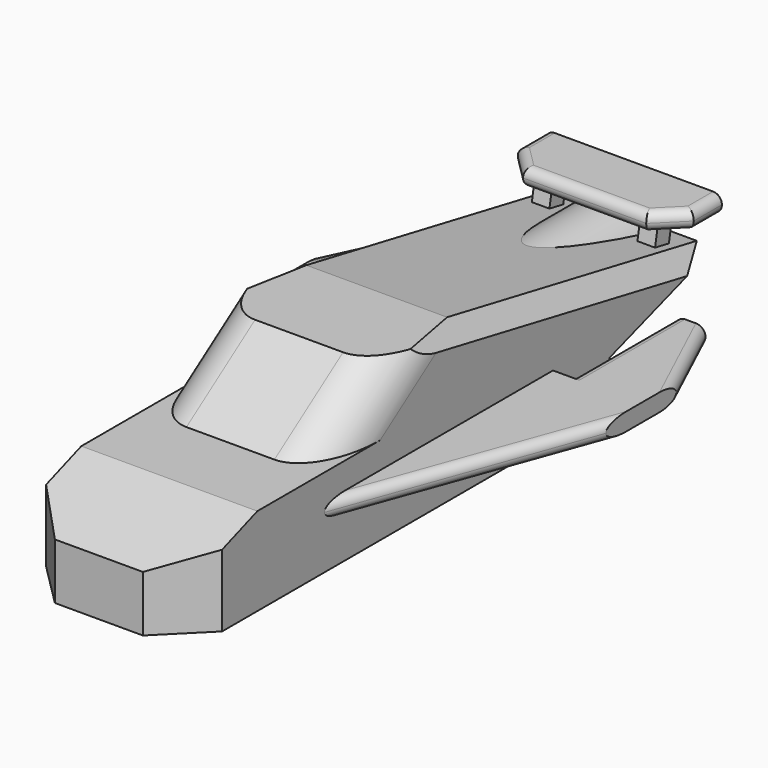
from build123d import *

# Parameters (mm, degrees)
F1_DEPTH     = 10
F2_DEPTH     = 10
F3_R         = 5
F4_T1_DEPTH  = 71.883894651
F5_T1_DEPTH  = 56.6843134125
F6_SIZE      = 3
F7_SIZE      = 5
F10_DEPTH    = 10
F9_W         = 35
F9_H         = 2
F11_DEPTH    = 10
F12_T4_DEPTH = 157.651683953
F13_T4_DEPTH = 157.651683953
F14_W        = 8
F14_H        = 2
F15_W        = 8
F15_H        = 2
F16_DEPTH    = 15
F17_SIZE2    = 4.6630765815
F17_SIZE     = 10
F18_SIZE2    = 4.6630765815
F18_SIZE     = 10
F19_R        = 0.99999
F20_R        = 5
F21_DEPTH    = 45
F22_R        = 2.9781353661
F23_DEPTH    = 5
F25_W        = 2
F25_H        = 2
F26_DEPTH    = 4
F28_DEPTH    = 15
F29_DEPTH    = 5
F30_W        = 5
F30_H        = 2
F31_DEPTH    = 2
F32_SIZE     = 3
F33_R        = 0.99999


# Not quite as in the source:
# - a fillet or chamfer that OpenCascade refuses, or shapes differently, is made with other operations: its cross-section is extruded or revolved along the edge and cut away or added
# - a fillet or chamfer is up to 0.001 mm smaller than in the source, because OpenCascade refuses the exact size


with BuildPart() as f1:
    # F0 (on Right) → F1 (new body)
    with BuildSketch(Plane.YZ):
        Polygon((30, 5), (30, 0), (44.9290536344, 5), (9.4593074173, 11.7742568254), (-1.5650746645, 11.7742568254), (-11.31126564, 5), align=None)
        Polygon((30, 0), (0, 0), (-30, 0), (-30, -5), (30, -5), align=None)
        Polygon((-30, 0), (0, 0), (30, 0), (30, 5), (-11.31126564, 5), (-30, 5), align=None)
    extrude(amount=-F1_DEPTH)

    # F2 (add): a face of the model
    f2_faces = [f1.faces().sort_by_distance(p)[0] for p in [
        (0, 4.6213303299, 2.1526362718),
    ]]
    extrude(f2_faces, amount=F2_DEPTH)

    # F3
    f3_edges = [f1.edges().sort_by_distance(p)[0] for p in [
        (-10, -6.43817, 8.387128),
        (10, -6.43817, 8.387128),
    ]]
    fillet(f3_edges, radius=F3_R)

    # F4: chamfer of 10 x 3.6397023427 on 1 edges, made by hand

    # F4_s2 → F4_t1 (cut)
    with BuildSketch(Plane.YZ.offset(-35.9419473255)):
        Polygon((-20, 5), (-30, 1.3602976573), (-30, 5), align=None)
    extrude(amount=F4_T1_DEPTH, mode=Mode.SUBTRACT)

    # F5: chamfer of 2 on 2 edges, made by hand

    # F5_s2 → F5_t1 (cut)
    with BuildSketch(Plane(origin=(0, 47.4786197454, -9.0677943367), x_dir=(1, 0, 0), z_dir=(0, -0.9822462418, 0.1875961634))):
        Polygon((-10, 11.3397492965), (-8, 13.3397492965), (-10, 13.3397492965), align=None)
        Polygon((10, 11.3397492965), (8, 13.3397492965), (10, 13.3397492965), align=None)
    extrude(amount=F5_T1_DEPTH, mode=Mode.SUBTRACT)

    # F6
    f6_edges = [f1.edges().sort_by_distance(p)[0] for p in [
        (0, 30, -5),
    ]]
    chamfer(f6_edges, length=F6_SIZE)

    # F7
    f7_edges = [f1.edges().sort_by_distance(p)[0] for p in [
        (-10, -30, -1.819851),
        (10, -30, -1.819851),
    ]]
    chamfer(f7_edges, length=F7_SIZE)

    # F8 (on face) → F10 (join)
    with BuildSketch(Plane.YZ.offset(10)):
        Polygon((-13, 0), (0, 0), (22, 0), (22, 2), (-13, 2), align=None)
    extrude(amount=F10_DEPTH)

    # F9 (on face) → F11 (join)
    with BuildSketch(Plane(origin=(-10, 0, 0), x_dir=(0, -1, 0), z_dir=(-1, 0, 0))):
        with Locations((-4.5269672573, 1)):
            Rectangle(F9_W, F9_H)
    extrude(amount=F11_DEPTH)

    # F12: chamfer of 30 x 10.919107028 on 1 edges, made by hand


with BuildPart() as f12_tool2:
    # F12_s3 → F12_t4 (new body)
    with BuildSketch(Plane.XY.offset(-77.8258419765)):
        Polygon((-9.080892972, -12.9730327427), (-20, 17.0269672573), (-20, -12.9730327427), align=None)
    extrude(amount=F12_T4_DEPTH)

    split(bisect_by=Plane.YZ.offset(-10), keep=Keep.BOTTOM)


with BuildPart() as f1_1:
    add(f1.part)

    # F12_t1: cut F12_tool2
    add(f12_tool2.part, mode=Mode.SUBTRACT)

    # F13: chamfer of 30 x 10.919107028 on 1 edges, made by hand


with BuildPart() as f13_tool2:
    # F13_s3 → F13_t4 (new body)
    with BuildSketch(Plane.XY.offset(79.8258419765)):
        Polygon((9.080892972, -13), (20, 17), (20, -13), align=None)
    extrude(amount=-F13_T4_DEPTH)

    split(bisect_by=Plane.YZ.offset(10), keep=Keep.TOP)


with BuildPart() as f1_2:
    add(f1_1.part)

    # F13_t1: cut F13_tool2
    add(f13_tool2.part, mode=Mode.SUBTRACT)

    # F14 (on face) + F15 (on face) → F16 (join)
    with BuildSketch(Plane(origin=(0, 22, 0), x_dir=(-1, 0, 0), z_dir=(0, 1, 0))):
        with Locations((-16, 1)):
            Rectangle(F14_W, F14_H)
    with BuildSketch(Plane(origin=(0, 22.0269672573, 0), x_dir=(-1, 0, 0), z_dir=(0, 1, 0))):
        with Locations((16, 1)):
            Rectangle(F15_W, F15_H)
    extrude(amount=F16_DEPTH)

    # F17
    f17_edges = [f1_2.edges().sort_by_distance(p)[0] for p in [
        (20, 37, 1),
    ]]
    f17_side = f1_2.faces().sort_by_distance((20, 27, 1))[0]
    chamfer(f17_edges, length=F17_SIZE, length2=F17_SIZE2, reference=f17_side)

    # F18
    f18_edges = [f1_2.edges().sort_by_distance(p)[0] for p in [
        (-20, 37.026967, 1),
    ]]
    f18_side = f1_2.faces().sort_by_distance((-20, 27.026967, 1))[0]
    chamfer(f18_edges, length=F18_SIZE, length2=F18_SIZE2, reference=f18_side)

    # F19 (radius 1 in the source; OpenCascade refuses exactly that, so slightly less here)
    f19_edges = [f1_2.edges().sort_by_distance(p)[0] for p in [
        (15, 3.262613, 2),
        (15, 3.262613, 0),
        (17.668462, 32, 0),
        (17.668462, 32, 2),
        (12, 29.5, 2),
        (12, 29.5, 0),
        (-15, 3.28958, 2),
        (-15, 3.28958, 0),
        (-17.668462, 32.026967, 2),
        (-12, 29.526967, 2),
        (-12, 29.526967, 0),
    ]]
    fillet(f19_edges, radius=F19_R)

    # F20 (on Front) → F21 (join)
    with BuildSketch(Plane.XZ):
        with Locations((0, 2.7116553392)):
            Circle(F20_R)
    extrude(amount=-F21_DEPTH)

    # F22 (on face) → F23 (cut)
    with BuildSketch(Plane(origin=(0, 45, 0), x_dir=(-1, 0, 0), z_dir=(0, 1, 0))):
        with Locations((0, 2.7116553392)):
            Circle(F22_R)
    extrude(amount=-F23_DEPTH, mode=Mode.SUBTRACT)

    # F24: chamfer of 2 on 1 edges, made by hand


with BuildPart() as f24_tool2:
    # F24_s3 → F24_t4 (revolve)
    with BuildSketch(Plane.XY.offset(2.7116553392)):
        Polygon((5, 43), (3, 45), (5, 45), align=None)
    revolve(axis=Axis((0, 45, 2.7116553392), (0, -1, 0)))

    split(bisect_by=Plane(origin=(0, 3.0256985599, -9.0341632165), x_dir=(1, 0, 0), z_dir=(0, 0.3175793108, -0.9482317129)), keep=Keep.TOP)


with BuildPart() as f1_3:
    add(f1_2.part)

    # F24_t1: cut F24_tool2
    add(f24_tool2.part, mode=Mode.SUBTRACT)


with BuildPart() as f24_tool7:
    # F24_s8 → F24_t9 (revolve)
    with BuildSketch(Plane.XY.offset(2.7116553392)):
        Polygon((5, 43), (3, 45), (5, 45), align=None)
    revolve(axis=Axis((0, 45, 2.7116553392), (0, -1, 0)))

    split(bisect_by=Plane(origin=(0, 2.5024857889, 13.1029186126), x_dir=(1, 0, 0), z_dir=(0, 0.1875961634, 0.9822462418)), keep=Keep.TOP)


with BuildPart() as f1_4:
    add(f1_3.part)

    # F24_t6: cut F24_tool7
    add(f24_tool7.part, mode=Mode.SUBTRACT)

    # F25 (on face) → F26 (join)
    with BuildSketch(Plane(origin=(0, 2.5024857889, 13.1029186126), x_dir=(1, 0, 0), z_dir=(0, 0.1875961634, 0.9822462418))):
        with Locations((-6, 39.4243540466)):
            Rectangle(F25_W, F25_H)
        with Locations((6, 39.4243540466)):
            Rectangle(F25_W, F25_H)
    extrude(amount=F26_DEPTH)

    # F27 (on face) → F28 (join)
    with BuildSketch(Plane(origin=(5, 0, 0), x_dir=(0, -1, 0), z_dir=(-1, 0, 0))):
        Polygon((-42.9595402808, 9.4484498521), (-40.9950477973, 9.8236421789), (-45.9950477973, 9.8236421789), (-45.9950477973, 7.8236421789), (-42.6492233025, 7.8236421789), align=None)
        Polygon((-40.9950477973, 7.8236421789), (-40.9950477973, 9.8236421789), (-42.9595402808, 9.4484498521), (-42.6492233025, 7.8236421789), align=None)
    extrude(amount=F28_DEPTH)

    # F27 (on face) → F29 (join)
    with BuildSketch(Plane(origin=(5, 0, 0), x_dir=(0, -1, 0), z_dir=(-1, 0, 0))):
        Polygon((-42.9595402808, 9.4484498521), (-40.9950477973, 9.8236421789), (-45.9950477973, 9.8236421789), (-45.9950477973, 7.8236421789), (-42.6492233025, 7.8236421789), align=None)
        Polygon((-40.9950477973, 7.8236421789), (-40.9950477973, 9.8236421789), (-42.9595402808, 9.4484498521), (-42.6492233025, 7.8236421789), align=None)
    extrude(amount=-F29_DEPTH)

    # F30 (on face) → F31 (join)
    with BuildSketch(Plane.XZ.offset(-40.9950477973)):
        with Locations((-7.5, 8.8236421789)):
            Rectangle(F30_W, F30_H)
        Polygon((-5, 7.8236421789), (0, 7.8236421789), (5, 7.8236421789), (5, 9.8236421789), (0, 9.8236421789), (-5, 9.8236421789), align=None)
        with Locations((7.5, 8.8236421789)):
            Rectangle(F30_W, F30_H)
    extrude(amount=F31_DEPTH)

    # F32
    f32_edges = [f1_4.edges().sort_by_distance(p)[0] for p in [
        (-10, 38.995048, 8.823642),
        (10, 38.995048, 8.823642),
    ]]
    chamfer(f32_edges, length=F32_SIZE)

    # F33 (radius 1 in the source; OpenCascade refuses exactly that, so slightly less here)
    f33_edges = [f1_4.edges().sort_by_distance(p)[0] for p in [
        (0, 38.995048, 7.823642),
        (0, 38.995048, 9.823642),
        (-8.5, 40.495048, 9.823642),
        (-8.5, 40.495048, 7.823642),
        (8.5, 40.495048, 9.823642),
        (8.5, 40.495048, 7.823642),
        (10, 43.995048, 7.823642),
        (10, 43.995048, 9.823642),
        (-10, 43.995048, 9.823642),
        (-10, 43.995048, 7.823642),
    ]]
    fillet(f33_edges, radius=F33_R)


solid = f1_4.part
